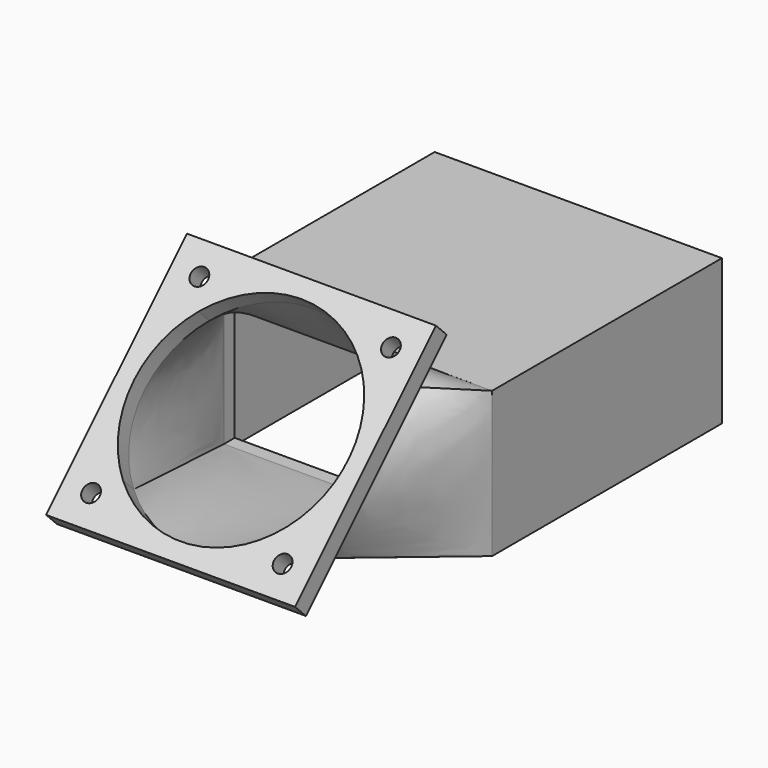
from build123d import *

# Parameters (mm, degrees)
F1_W      = 75
F1_H      = 75
F2_DEPTH  = 38
F3_W      = 68
F3_H      = 68
F4_DEPTH  = 35
F6_W      = 65
F6_H      = 32
F7_DEPTH  = 75
F9_W      = 65
F9_H      = 32
F10_W     = 75
F10_H     = 38
F18_DEPTH = 5
F21_R     = 2.25
F22_DEPTH = 5
F19_W     = 65
F19_H     = 65
F23_DEPTH = 5


# Not quite as in the source:
# - a feature of the source that left no trace in its solid (it failed there, or was rolled back) is left out
# - the arcs of a loft's sections are written as splines that run evenly, so that the points pair up as in the source's solid


with BuildPart() as f2:
    # F1 (on offset) → F2 (new body)
    with BuildSketch(Plane.XY.offset(3)):
        Rectangle(F1_W, F1_H)
    extrude(amount=-F2_DEPTH)


with BuildPart() as f4:
    # F3 (on Top) → F4 (new body, through all)
    with BuildSketch(Plane.XY):
        Rectangle(F3_W, F3_H)
    extrude(amount=-F4_DEPTH)


with BuildPart() as f2_1:
    add(f2.part)

    # F5: cut F4
    add(f4.part, mode=Mode.SUBTRACT)


with BuildPart() as f7:
    # F6 (on face) → F7 (new body, through all)
    with BuildSketch(Plane.XZ.offset(37.5)):
        with Locations((0, -16)):
            Rectangle(F6_W, F6_H)
    extrude(amount=-F7_DEPTH)


with BuildPart() as f2_2:
    add(f2_1.part)

    # F8: cut F7
    add(f7.part, mode=Mode.SUBTRACT)


with BuildPart() as f15:
    # F9 (on face) → F15 section 0
    with BuildSketch(Plane.XZ.offset(37.5)):
        with Locations((0, -16)):
            Rectangle(F9_W, F9_H)
    # F14 (on offset) → F15 section 1
    with BuildSketch(Plane(origin=(0, -31.8921356237, 31.8921356237), x_dir=(-1, 0, 0), z_dir=(0, 0.7071067812, -0.7071067812))):
        with BuildLine():
            ThreePointArc((19.3777270669, -72.7305613051), (27.9634183298, -53.9499033063), (21.3394636211, -34.3910067794))
            ThreePointArc((21.3394636211, -34.3910067794), (0.2969683656, -24.5206618662), (-20.9501510919, -33.9424573448))
            ThreePointArc((-20.9501510919, -33.9424573448), (-27.8904955693, -54.9930022936), (-17.3532530257, -74.4932675145))
            ThreePointArc((-17.3532530257, -74.4932675145), (1.3421650722, -80.4869005137), (19.3777270669, -72.7305613051))
        make_face()
    loft()


with BuildPart() as f17:
    # F10 (on face) → F17 section 0
    with BuildSketch(Plane.XZ.offset(37.5)):
        with Locations((0, -16)):
            Rectangle(F10_W, F10_H)
    # F16 (on offset) → F17 section 1
    with BuildSketch(Plane(origin=(0, -31.8921356237, 31.8921356237), x_dir=(-1, 0, 0), z_dir=(0, 0.7071067812, -0.7071067812))):
        with BuildLine():
            add(Edge.make_bspline(
                [(-24.0003369849, -34.5195363186), (-25.1784048219, -36.090354701), (-26.2017352476, -37.7771609273), (-27.8996955072, -41.31809129), (-28.5742833559, -43.1721278699), (-29.5488165406, -46.9762758623), (-29.8487377794, -48.9262932099), (-30.0623931254, -52.8474675582), (-29.9761219495, -54.8185276002), (-29.4206888016, -58.7060397732), (-28.9515405638, -60.6223957777), (-27.6483639065, -64.3268508627), (-26.8143677105, -66.1148583431), (-24.8135278918, -69.4938962086), (-23.6467337438, -71.0848430403), (-21.0251219159, -74.0086091562), (-19.5703690605, -75.3413561445), (-17.9995506781, -76.5194239816)],
                knots=[0, 0, 0, 0, 0.125, 0.125, 0.25, 0.25, 0.375, 0.375, 0.5, 0.5, 0.625, 0.625, 0.75, 0.75, 0.875, 0.875, 1, 1, 1, 1], degree=3))
            add(Edge.make_bspline(
                [(-17.9995506781, -76.5194239816), (-16.4287322957, -77.6974918186), (-14.7419260694, -78.7208222443), (-11.2009957067, -80.418782504), (-9.3469591268, -81.0933703526), (-5.5428111344, -82.0679035373), (-3.5927937869, -82.3678247761), (0.3283805615, -82.5814801221), (2.2994406035, -82.4952089462), (6.1869527765, -81.9397757983), (8.103308781, -81.4706275605), (11.8077638659, -80.1674509032), (13.5957713464, -79.3334547072), (16.9748092119, -77.3326148885), (18.5657560436, -76.1658207405), (21.4895221595, -73.5442089126), (22.8222691478, -72.0894560572), (24.0003369849, -70.5186376748)],
                knots=[0, 0, 0, 0, 0.125, 0.125, 0.25, 0.25, 0.375, 0.375, 0.5, 0.5, 0.625, 0.625, 0.75, 0.75, 0.875, 0.875, 1, 1, 1, 1], degree=3))
            add(Edge.make_bspline(
                [(24.0003369849, -70.5186376748), (25.1784048219, -68.9478192924), (26.2017352476, -67.2610130661), (27.8996955072, -63.7200827034), (28.5742833559, -61.8660461235), (29.5488165406, -58.0618981311), (29.8487377794, -56.1118807836), (30.0623931254, -52.1907064353), (29.9761219495, -50.2196463932), (29.4206888016, -46.3321342203), (28.9515405638, -44.4157782157), (27.6483639065, -40.7113231308), (26.8143677105, -38.9233156503), (24.8135278918, -35.5442777848), (23.6467337438, -33.9533309531), (21.0251219159, -31.0295648372), (19.5703690605, -29.6968178489), (17.9995506781, -28.5187500119)],
                knots=[0, 0, 0, 0, 0.125, 0.125, 0.25, 0.25, 0.375, 0.375, 0.5, 0.5, 0.625, 0.625, 0.75, 0.75, 0.875, 0.875, 1, 1, 1, 1], degree=3))
            add(Edge.make_bspline(
                [(17.9995506781, -28.5187500119), (16.4287322957, -27.3406821748), (14.7419260694, -26.3173517491), (11.2009957067, -24.6193914895), (9.3469591268, -23.9448036409), (5.5428111344, -22.9702704561), (3.5927937869, -22.6703492173), (-0.3283805615, -22.4566938713), (-2.2994406035, -22.5429650472), (-6.1869527765, -23.0983981951), (-8.103308781, -23.5675464329), (-11.8077638659, -24.8707230902), (-13.5957713464, -25.7047192862), (-16.9748092119, -27.7055591049), (-18.5657560436, -28.8723532529), (-21.4895221595, -31.4939650809), (-22.8222691478, -32.9487179362), (-24.0003369849, -34.5195363186)],
                knots=[0, 0, 0, 0, 0.125, 0.125, 0.25, 0.25, 0.375, 0.375, 0.5, 0.5, 0.625, 0.625, 0.75, 0.75, 0.875, 0.875, 1, 1, 1, 1], degree=3))
        make_face()
    loft(ruled=True)

    # F25: cut F15
    add(f15.part, mode=Mode.SUBTRACT)


with BuildPart() as f18:
    # F14 (on offset) → F18 (new body)
    with BuildSketch(Plane(origin=(0, -31.8921356237, 31.8921356237), x_dir=(-1, 0, 0), z_dir=(0, 0.7071067812, -0.7071067812))):
        with BuildLine():
            ThreePointArc((19.3777270669, -72.7305613051), (27.9634183298, -53.9499033063), (21.3394636211, -34.3910067794))
            ThreePointArc((21.3394636211, -34.3910067794), (0.2969683656, -24.5206618662), (-20.9501510919, -33.9424573448))
            ThreePointArc((-20.9501510919, -33.9424573448), (-27.8904955693, -54.9930022936), (-17.3532530257, -74.4932675145))
            ThreePointArc((-17.3532530257, -74.4932675145), (1.3421650722, -80.4869005137), (19.3777270669, -72.7305613051))
        make_face()
    extrude(amount=-F18_DEPTH)


with BuildPart() as f22:
    # F21 (on face) → F22 (new body)
    with BuildSketch(Plane(origin=(0, -31.8921356237, 31.8921356237), x_dir=(-1, 0, 0), z_dir=(0, 0.7071067812, -0.7071067812))):
        with Locations((-25, -27.5190869967)):
            Circle(F21_R)
    extrude(amount=-F22_DEPTH)


with BuildPart() as f22b:
    # F21 (on face) → F22, piece 2 (new body)
    with BuildSketch(Plane(origin=(0, -31.8921356237, 31.8921356237), x_dir=(-1, 0, 0), z_dir=(0, 0.7071067812, -0.7071067812))):
        with Locations((25, -27.5190869967)):
            Circle(F21_R)
    extrude(amount=-F22_DEPTH)


with BuildPart() as f22c:
    # F21 (on face) → F22, piece 3 (new body)
    with BuildSketch(Plane(origin=(0, -31.8921356237, 31.8921356237), x_dir=(-1, 0, 0), z_dir=(0, 0.7071067812, -0.7071067812))):
        with Locations((25, -77.5190869967)):
            Circle(F21_R)
    extrude(amount=-F22_DEPTH)


with BuildPart() as f22d:
    # F21 (on face) → F22, piece 4 (new body)
    with BuildSketch(Plane(origin=(0, -31.8921356237, 31.8921356237), x_dir=(-1, 0, 0), z_dir=(0, 0.7071067812, -0.7071067812))):
        with Locations((-25, -77.5190869967)):
            Circle(F21_R)
    extrude(amount=-F22_DEPTH)


with BuildPart() as f23:
    # F19 (on offset) → F23 (new body)
    with BuildSketch(Plane(origin=(0, -31.8921356237, 31.8921356237), x_dir=(-1, 0, 0), z_dir=(0, 0.7071067812, -0.7071067812))):
        with Locations((0, -52.5190869967)):
            Rectangle(F19_W, F19_H)
    extrude(amount=-F23_DEPTH)

    # F24: cut F22, F22b, F22c, F22d, F18
    add(f22.part, mode=Mode.SUBTRACT)
    add(f22b.part, mode=Mode.SUBTRACT)
    add(f22c.part, mode=Mode.SUBTRACT)
    add(f22d.part, mode=Mode.SUBTRACT)
    add(f18.part, mode=Mode.SUBTRACT)


solid = Compound([f2_2.part, f17.part, f23.part])
